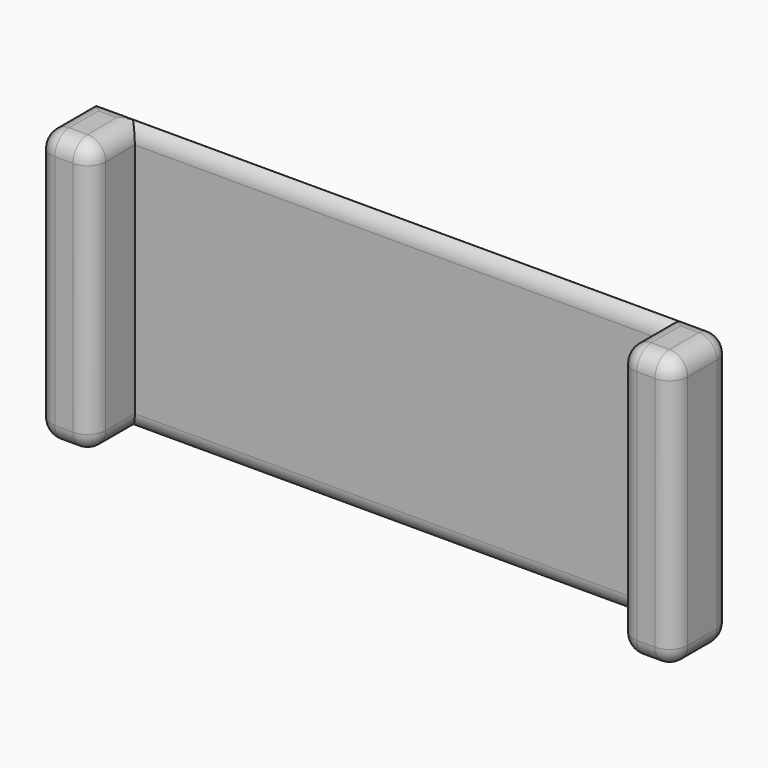
from build123d import *

# Parameters (mm, degrees)
F0_W          = 350
F0_H          = 150
F1_DEPTH      = 10
F2_W          = 30
F2_H          = 150
F3_DEPTH      = 40
F4_T1_DEPTH   = 10
F4_T3_DEPTH   = 20
F4_T5_DEPTH   = 130
F4_T7_DEPTH   = 55
F4_T9_DEPTH   = 365
F4_T11_DEPTH  = 290
F4_T13_DEPTH  = 10
F4_S17_W      = 10.2
F4_S17_H      = 10.2
F4_T18_DEPTH  = 10.2
F4_S23_W      = 10.2
F4_S23_H      = 10.2
F4_T24_DEPTH  = 10.2
F4_S29_W      = 10.2
F4_S29_H      = 10.2
F4_T30_DEPTH  = 10.2
F4_S35_W      = 10.2
F4_S35_H      = 10.2
F4_T36_DEPTH  = 10.2
F4_S41_W      = 10.2
F4_S41_H      = 10.2
F4_T42_DEPTH  = 10.2
F4_S47_W      = 10.2
F4_S47_H      = 10.2
F4_T48_DEPTH  = 10.2
F4_S53_W      = 10.2
F4_S53_H      = 10.2
F4_T54_DEPTH  = 10.2
F4_S59_W      = 10.2
F4_S59_H      = 10.2
F4_T60_DEPTH  = 10.2
F4_S65_W      = 10.2
F4_S65_H      = 10.2
F4_T66_DEPTH  = 10.2
F4_S71_W      = 10.2
F4_S71_H      = 10.2
F4_T72_DEPTH  = 10.2
F4_T79_DEPTH  = 45
F4_T84_DEPTH  = 315
F4_T91_DEPTH  = 315
F4_T95_DEPTH  = 45
F4_T103_DEPTH = 45
F4_T108_DEPTH = 315
F4_T115_DEPTH = 315
F4_T119_DEPTH = 45


# Not quite as in the source:
# - a fillet or chamfer that OpenCascade refuses, or shapes differently, is made with other operations: its cross-section is extruded or revolved along the edge and cut away or added


with BuildPart() as f1:
    # F0 (on Front) → F1 (new body)
    with BuildSketch(Plane.XZ):
        Rectangle(F0_W, F0_H)
    extrude(amount=F1_DEPTH)

    # F2 (on face) → F3 (join)
    with BuildSketch(Plane(origin=(0, 0, 0), x_dir=(-1, 0, 0), z_dir=(0, 1, 0))):
        with Locations((-160, 0)):
            Rectangle(F2_W, F2_H)
        with Locations((160, 0)):
            Rectangle(F2_W, F2_H)
    extrude(amount=-F3_DEPTH)

    # F4: fillet of radius 10 on 21 edges, made by hand

    # F4_s2 → F4_t1 (cut)
    with BuildSketch(Plane.YZ.offset(155)):
        with BuildLine():
            ThreePointArc((-30, 75), (-37.0710678119, 72.0710678119), (-40, 65))
            Line((-40, 65), (-40, 75))
            Line((-40, 75), (-30, 75))
        make_face()
        with BuildLine():
            ThreePointArc((-30, -75), (-37.0710678119, -72.0710678119), (-40, -65))
            Line((-40, -65), (-40, -75))
            Line((-40, -75), (-30, -75))
        make_face()
    extrude(amount=F4_T1_DEPTH, mode=Mode.SUBTRACT)

    # F4_s4 → F4_t3 (cut)
    with BuildSketch(Plane.XZ.offset(10)):
        with BuildLine():
            ThreePointArc((155, 75), (147.9289321881, 72.0710678119), (145, 65))
            Line((145, 65), (145, 75))
            Line((145, 75), (155, 75))
        make_face()
        with BuildLine():
            ThreePointArc((165, -75), (172.0710678119, -72.0710678119), (175, -65))
            Line((175, -65), (175, -75))
            Line((175, -75), (165, -75))
        make_face()
        with BuildLine():
            ThreePointArc((155, -75), (147.9289321881, -72.0710678119), (145, -65))
            Line((145, -65), (145, -75))
            Line((145, -75), (155, -75))
        make_face()
        with BuildLine():
            ThreePointArc((175, 65), (172.0710678119, 72.0710678119), (165, 75))
            Line((165, 75), (175, 75))
            Line((175, 75), (175, 65))
        make_face()
        with BuildLine():
            ThreePointArc((-155, -75), (-147.9289321881, -72.0710678119), (-145, -65))
            Line((-145, -65), (-145, -75))
            Line((-145, -75), (-155, -75))
        make_face()
        with BuildLine():
            ThreePointArc((-155, 75), (-147.9289321881, 72.0710678119), (-145, 65))
            Line((-145, 65), (-145, 75))
            Line((-145, 75), (-155, 75))
        make_face()
    extrude(amount=F4_T3_DEPTH, mode=Mode.SUBTRACT)

    # F4_s6 → F4_t5 (cut)
    with BuildSketch(Plane.XY.offset(-65)):
        with BuildLine():
            ThreePointArc((175, -30), (172.0710678119, -37.0710678119), (165, -40))
            Line((165, -40), (175, -40))
            Line((175, -40), (175, -30))
        make_face()
        with BuildLine():
            ThreePointArc((175, -10), (172.0710678119, -2.9289321881), (165, 0))
            Line((165, 0), (175, 0))
            Line((175, 0), (175, -10))
        make_face()
        with BuildLine():
            ThreePointArc((-165, -40), (-172.0710678119, -37.0710678119), (-175, -30))
            Line((-175, -30), (-175, -40))
            Line((-175, -40), (-165, -40))
        make_face()
        with BuildLine():
            ThreePointArc((155, -40), (147.9289321881, -37.0710678119), (145, -30))
            Line((145, -30), (145, -40))
            Line((145, -40), (155, -40))
        make_face()
        with BuildLine():
            ThreePointArc((-145, -30), (-147.9289321881, -37.0710678119), (-155, -40))
            Line((-155, -40), (-145, -40))
            Line((-145, -40), (-145, -30))
        make_face()
    extrude(amount=F4_T5_DEPTH, mode=Mode.SUBTRACT)

    # F4_s8 → F4_t7 (cut)
    with BuildSketch(Plane.XZ.offset(-25)):
        with BuildLine():
            ThreePointArc((-165, -75), (-172.0710678119, -72.0710678119), (-175, -65))
            Line((-175, -65), (-175, -75))
            Line((-175, -75), (-165, -75))
        make_face()
        with BuildLine():
            ThreePointArc((-165, 75), (-172.0710678119, 72.0710678119), (-175, 65))
            Line((-175, 65), (-175, 75))
            Line((-175, 75), (-165, 75))
        make_face()
    extrude(amount=F4_T7_DEPTH, mode=Mode.SUBTRACT)

    # F4_s10 → F4_t9 (cut)
    with BuildSketch(Plane.YZ.offset(-200)):
        with BuildLine():
            ThreePointArc((-10, 75), (-2.9289321881, 72.0710678119), (0, 65))
            Line((0, 65), (0, 75))
            Line((0, 75), (-10, 75))
        make_face()
        with BuildLine():
            ThreePointArc((-10, -75), (-2.9289321881, -72.0710678119), (0, -65))
            Line((0, -65), (0, -75))
            Line((0, -75), (-10, -75))
        make_face()
    extrude(amount=F4_T9_DEPTH, mode=Mode.SUBTRACT)

    # F4_s12 → F4_t11 (cut)
    with BuildSketch(Plane.YZ.offset(-145)):
        with BuildLine():
            ThreePointArc((0, 75), (-7.0710678119, 72.0710678119), (-10, 65))
            Line((-10, 65), (-10, 75))
            Line((-10, 75), (0, 75))
        make_face()
        with BuildLine():
            ThreePointArc((0, -75), (-7.0710678119, -72.0710678119), (-10, -65))
            Line((-10, -65), (-10, -75))
            Line((-10, -75), (0, -75))
        make_face()
    extrude(amount=F4_T11_DEPTH, mode=Mode.SUBTRACT)

    # F4_s14 → F4_t13 (cut)
    with BuildSketch(Plane.YZ.offset(-165)):
        with BuildLine():
            ThreePointArc((-30, 75), (-37.0710678119, 72.0710678119), (-40, 65))
            Line((-40, 65), (-40, 75))
            Line((-40, 75), (-30, 75))
        make_face()
        with BuildLine():
            ThreePointArc((-30, -75), (-37.0710678119, -72.0710678119), (-40, -65))
            Line((-40, -65), (-40, -75))
            Line((-40, -75), (-30, -75))
        make_face()
    extrude(amount=F4_T13_DEPTH, mode=Mode.SUBTRACT)


with BuildPart() as f4_tool16:
    # F4_s17 → F4_t18 (new body)
    with BuildSketch(Plane.XY.offset(65)):
        with Locations((149.9, -35.1)):
            Rectangle(F4_S17_W, F4_S17_H)
    extrude(amount=F4_T18_DEPTH)

    # F4_s19 → F4_t20 (revolve, cut)
    with BuildSketch(Plane(origin=(155, -30, 65), x_dir=(0.7071067812, 0.7071067812, 0), z_dir=(0.7071067812, -0.7071067812, 0))):
        with BuildLine():
            ThreePointArc((0, -10), (10, 0), (0, 10))
            Line((0, 10), (0, -10))
        make_face()
    revolve(axis=Axis((155, -30, 65), (0, 0, 1)), mode=Mode.SUBTRACT)


with BuildPart() as f1_1:
    add(f1.part)

    # F4_t15: cut F4_tool16
    add(f4_tool16.part, mode=Mode.SUBTRACT)


with BuildPart() as f4_tool22:
    # F4_s23 → F4_t24 (new body)
    with BuildSketch(Plane.YZ.offset(165)):
        with Locations((-35.1, 70.1)):
            Rectangle(F4_S23_W, F4_S23_H)
    extrude(amount=F4_T24_DEPTH)

    # F4_s25 → F4_t26 (revolve, cut)
    with BuildSketch(Plane(origin=(165, -30, 65), x_dir=(0, 0.7071067812, -0.7071067812), z_dir=(0, -0.7071067812, -0.7071067812))):
        with BuildLine():
            ThreePointArc((0, -10), (10, 0), (0, 10))
            Line((0, 10), (0, -10))
        make_face()
    revolve(axis=Axis((165, -30, 65), (1, 0, 0)), mode=Mode.SUBTRACT)


with BuildPart() as f1_2:
    add(f1_1.part)

    # F4_t21: cut F4_tool22
    add(f4_tool22.part, mode=Mode.SUBTRACT)


with BuildPart() as f4_tool28:
    # F4_s29 → F4_t30 (new body)
    with BuildSketch(Plane.XY.offset(-65)):
        with Locations((170.1, -4.9)):
            Rectangle(F4_S29_W, F4_S29_H)
    extrude(amount=-F4_T30_DEPTH)

    # F4_s31 → F4_t32 (revolve, cut)
    with BuildSketch(Plane(origin=(165, -10, -65), x_dir=(-0.7071067812, -0.7071067812, 0), z_dir=(0.7071067812, -0.7071067812, 0))):
        with BuildLine():
            ThreePointArc((0, -10), (10, 0), (0, 10))
            Line((0, 10), (0, -10))
        make_face()
    revolve(axis=Axis((165, -10, -65), (0, 0, -1)), mode=Mode.SUBTRACT)


with BuildPart() as f1_3:
    add(f1_2.part)

    # F4_t27: cut F4_tool28
    add(f4_tool28.part, mode=Mode.SUBTRACT)


with BuildPart() as f4_tool34:
    # F4_s35 → F4_t36 (new body)
    with BuildSketch(Plane.XY.offset(-65)):
        with Locations((170.1, -35.1)):
            Rectangle(F4_S35_W, F4_S35_H)
    extrude(amount=-F4_T36_DEPTH)

    # F4_s37 → F4_t38 (revolve, cut)
    with BuildSketch(Plane(origin=(165, -30, -65), x_dir=(-0.7071067812, 0.7071067812, 0), z_dir=(-0.7071067812, -0.7071067812, 0))):
        with BuildLine():
            ThreePointArc((0, -10), (10, 0), (0, 10))
            Line((0, 10), (0, -10))
        make_face()
    revolve(axis=Axis((165, -30, -65), (0, 0, -1)), mode=Mode.SUBTRACT)


with BuildPart() as f1_4:
    add(f1_3.part)

    # F4_t33: cut F4_tool34
    add(f4_tool34.part, mode=Mode.SUBTRACT)


with BuildPart() as f4_tool40:
    # F4_s41 → F4_t42 (new body)
    with BuildSketch(Plane.XY.offset(-65)):
        with Locations((149.9, -35.1)):
            Rectangle(F4_S41_W, F4_S41_H)
    extrude(amount=-F4_T42_DEPTH)

    # F4_s43 → F4_t44 (revolve, cut)
    with BuildSketch(Plane(origin=(155, -30, -65), x_dir=(0.7071067812, 0.7071067812, 0), z_dir=(-0.7071067812, 0.7071067812, 0))):
        with BuildLine():
            ThreePointArc((0, -10), (10, 0), (0, 10))
            Line((0, 10), (0, -10))
        make_face()
    revolve(axis=Axis((155, -30, -65), (0, 0, -1)), mode=Mode.SUBTRACT)


with BuildPart() as f1_5:
    add(f1_4.part)

    # F4_t39: cut F4_tool40
    add(f4_tool40.part, mode=Mode.SUBTRACT)


with BuildPart() as f4_tool46:
    # F4_s47 → F4_t48 (new body)
    with BuildSketch(Plane.YZ.offset(165)):
        with Locations((-4.9, 70.1)):
            Rectangle(F4_S47_W, F4_S47_H)
    extrude(amount=F4_T48_DEPTH)

    # F4_s49 → F4_t50 (revolve, cut)
    with BuildSketch(Plane(origin=(165, -10, 65), x_dir=(0, -0.7071067812, -0.7071067812), z_dir=(0, -0.7071067812, 0.7071067812))):
        with BuildLine():
            ThreePointArc((0, -10), (10, 0), (0, 10))
            Line((0, 10), (0, -10))
        make_face()
    revolve(axis=Axis((165, -10, 65), (1, 0, 0)), mode=Mode.SUBTRACT)


with BuildPart() as f1_6:
    add(f1_5.part)

    # F4_t45: cut F4_tool46
    add(f4_tool46.part, mode=Mode.SUBTRACT)


with BuildPart() as f4_tool52:
    # F4_s53 → F4_t54 (new body)
    with BuildSketch(Plane.XY.offset(-65)):
        with Locations((-149.9, -35.1)):
            Rectangle(F4_S53_W, F4_S53_H)
    extrude(amount=-F4_T54_DEPTH)

    # F4_s55 → F4_t56 (revolve, cut)
    with BuildSketch(Plane(origin=(-155, -30, -65), x_dir=(-0.7071067812, 0.7071067812, 0), z_dir=(-0.7071067812, -0.7071067812, 0))):
        with BuildLine():
            ThreePointArc((0, -10), (10, 0), (0, 10))
            Line((0, 10), (0, -10))
        make_face()
    revolve(axis=Axis((-155, -30, -65), (0, 0, -1)), mode=Mode.SUBTRACT)


with BuildPart() as f1_7:
    add(f1_6.part)

    # F4_t51: cut F4_tool52
    add(f4_tool52.part, mode=Mode.SUBTRACT)


with BuildPart() as f4_tool58:
    # F4_s59 → F4_t60 (new body)
    with BuildSketch(Plane.YZ.offset(-165)):
        with Locations((-35.1, -70.1)):
            Rectangle(F4_S59_W, F4_S59_H)
    extrude(amount=-F4_T60_DEPTH)

    # F4_s61 → F4_t62 (revolve, cut)
    with BuildSketch(Plane(origin=(-165, -30, -65), x_dir=(0, 0.7071067812, 0.7071067812), z_dir=(0, -0.7071067812, 0.7071067812))):
        with BuildLine():
            ThreePointArc((0, -10), (10, 0), (0, 10))
            Line((0, 10), (0, -10))
        make_face()
    revolve(axis=Axis((-165, -30, -65), (-1, 0, 0)), mode=Mode.SUBTRACT)


with BuildPart() as f1_8:
    add(f1_7.part)

    # F4_t57: cut F4_tool58
    add(f4_tool58.part, mode=Mode.SUBTRACT)


with BuildPart() as f4_tool64:
    # F4_s65 → F4_t66 (new body)
    with BuildSketch(Plane.YZ.offset(-165)):
        with Locations((-35.1, 70.1)):
            Rectangle(F4_S65_W, F4_S65_H)
    extrude(amount=-F4_T66_DEPTH)

    # F4_s67 → F4_t68 (revolve, cut)
    with BuildSketch(Plane(origin=(-165, -30, 65), x_dir=(0, 0.7071067812, -0.7071067812), z_dir=(0, 0.7071067812, 0.7071067812))):
        with BuildLine():
            ThreePointArc((0, -10), (10, 0), (0, 10))
            Line((0, 10), (0, -10))
        make_face()
    revolve(axis=Axis((-165, -30, 65), (-1, 0, 0)), mode=Mode.SUBTRACT)


with BuildPart() as f1_9:
    add(f1_8.part)

    # F4_t63: cut F4_tool64
    add(f4_tool64.part, mode=Mode.SUBTRACT)


with BuildPart() as f4_tool70:
    # F4_s71 → F4_t72 (new body)
    with BuildSketch(Plane.XY.offset(65)):
        with Locations((-149.9, -35.1)):
            Rectangle(F4_S71_W, F4_S71_H)
    extrude(amount=F4_T72_DEPTH)

    # F4_s73 → F4_t74 (revolve, cut)
    with BuildSketch(Plane(origin=(-155, -30, 65), x_dir=(-0.7071067812, 0.7071067812, 0), z_dir=(0.7071067812, 0.7071067812, 0))):
        with BuildLine():
            ThreePointArc((0, -10), (10, 0), (0, 10))
            Line((0, 10), (0, -10))
        make_face()
    revolve(axis=Axis((-155, -30, 65), (0, 0, 1)), mode=Mode.SUBTRACT)


with BuildPart() as f1_10:
    add(f1_9.part)

    # F4_t69: cut F4_tool70
    add(f4_tool70.part, mode=Mode.SUBTRACT)


with BuildPart() as f4_tool77:
    # F4_s78 → F4_t79 (new body)
    with BuildSketch(Plane.XZ.offset(-15)):
        with BuildLine():
            ThreePointArc((155, 75), (147.9289321881, 72.0710678119), (145, 65))
            Line((145, 65), (145, 75))
            Line((145, 75), (155, 75))
        make_face()
    extrude(amount=F4_T79_DEPTH)

    split(bisect_by=Plane.XZ.offset(10), keep=Keep.BOTTOM)

    split(bisect_by=Plane.XZ, keep=Keep.TOP)


with BuildPart() as f4_tool82:
    # F4_s83 → F4_t84 (new body)
    with BuildSketch(Plane.YZ.offset(170)):
        with BuildLine():
            ThreePointArc((0, 75), (-7.0710678119, 72.0710678119), (-10, 65))
            Line((-10, 65), (-10, 75))
            Line((-10, 75), (0, 75))
        make_face()
    extrude(amount=-F4_T84_DEPTH)

    split(bisect_by=Plane.YZ.offset(145), keep=Keep.TOP)


with BuildPart() as f4_tool77_1:
    add(f4_tool77.part)

    # F4_t86: intersect F4_tool82
    add(f4_tool82.part, mode=Mode.INTERSECT)


with BuildPart() as f1_11:
    add(f1_10.part)

    # F4_t75: cut F4_tool77
    add(f4_tool77_1.part, mode=Mode.SUBTRACT)


with BuildPart() as f4_tool89:
    # F4_s90 → F4_t91 (new body)
    with BuildSketch(Plane.YZ.offset(-145)):
        with BuildLine():
            ThreePointArc((0, -75), (-7.0710678119, -72.0710678119), (-10, -65))
            Line((-10, -65), (-10, -75))
            Line((-10, -75), (0, -75))
        make_face()
    extrude(amount=F4_T91_DEPTH)

    split(bisect_by=Plane.YZ.offset(145), keep=Keep.TOP)


with BuildPart() as f4_tool93:
    # F4_s94 → F4_t95 (new body)
    with BuildSketch(Plane.XZ.offset(-15)):
        with BuildLine():
            ThreePointArc((155, -75), (147.9289321881, -72.0710678119), (145, -65))
            Line((145, -65), (145, -75))
            Line((145, -75), (155, -75))
        make_face()
    extrude(amount=F4_T95_DEPTH)

    split(bisect_by=Plane.XZ.offset(10), keep=Keep.BOTTOM)

    split(bisect_by=Plane.XZ, keep=Keep.TOP)


with BuildPart() as f4_tool89_1:
    add(f4_tool89.part)

    # F4_t98: intersect F4_tool93
    add(f4_tool93.part, mode=Mode.INTERSECT)


with BuildPart() as f1_12:
    add(f1_11.part)

    # F4_t87: cut F4_tool89
    add(f4_tool89_1.part, mode=Mode.SUBTRACT)


with BuildPart() as f4_tool101:
    # F4_s102 → F4_t103 (new body)
    with BuildSketch(Plane.XZ.offset(-15)):
        with BuildLine():
            ThreePointArc((-155, -75), (-147.9289321881, -72.0710678119), (-145, -65))
            Line((-145, -65), (-145, -75))
            Line((-145, -75), (-155, -75))
        make_face()
    extrude(amount=F4_T103_DEPTH)

    split(bisect_by=Plane.XZ.offset(10), keep=Keep.BOTTOM)

    split(bisect_by=Plane.XZ, keep=Keep.TOP)


with BuildPart() as f4_tool106:
    # F4_s107 → F4_t108 (new body)
    with BuildSketch(Plane.YZ.offset(-170)):
        with BuildLine():
            ThreePointArc((0, -75), (-7.0710678119, -72.0710678119), (-10, -65))
            Line((-10, -65), (-10, -75))
            Line((-10, -75), (0, -75))
        make_face()
    extrude(amount=F4_T108_DEPTH)

    split(bisect_by=Plane.YZ.offset(-145), keep=Keep.BOTTOM)


with BuildPart() as f4_tool101_1:
    add(f4_tool101.part)

    # F4_t110: intersect F4_tool106
    add(f4_tool106.part, mode=Mode.INTERSECT)


with BuildPart() as f1_13:
    add(f1_12.part)

    # F4_t99: cut F4_tool101
    add(f4_tool101_1.part, mode=Mode.SUBTRACT)


with BuildPart() as f4_tool113:
    # F4_s114 → F4_t115 (new body)
    with BuildSketch(Plane.YZ.offset(145)):
        with BuildLine():
            ThreePointArc((0, 75), (-7.0710678119, 72.0710678119), (-10, 65))
            Line((-10, 65), (-10, 75))
            Line((-10, 75), (0, 75))
        make_face()
    extrude(amount=-F4_T115_DEPTH)

    split(bisect_by=Plane.YZ.offset(-145), keep=Keep.BOTTOM)


with BuildPart() as f4_tool117:
    # F4_s118 → F4_t119 (new body)
    with BuildSketch(Plane.XZ.offset(-15)):
        with BuildLine():
            ThreePointArc((-155, 75), (-147.9289321881, 72.0710678119), (-145, 65))
            Line((-145, 65), (-145, 75))
            Line((-145, 75), (-155, 75))
        make_face()
    extrude(amount=F4_T119_DEPTH)

    split(bisect_by=Plane.XZ.offset(10), keep=Keep.BOTTOM)

    split(bisect_by=Plane.XZ, keep=Keep.TOP)


with BuildPart() as f4_tool113_1:
    add(f4_tool113.part)

    # F4_t122: intersect F4_tool117
    add(f4_tool117.part, mode=Mode.INTERSECT)


with BuildPart() as f1_14:
    add(f1_13.part)

    # F4_t111: cut F4_tool113
    add(f4_tool113_1.part, mode=Mode.SUBTRACT)


solid = f1_14.part
